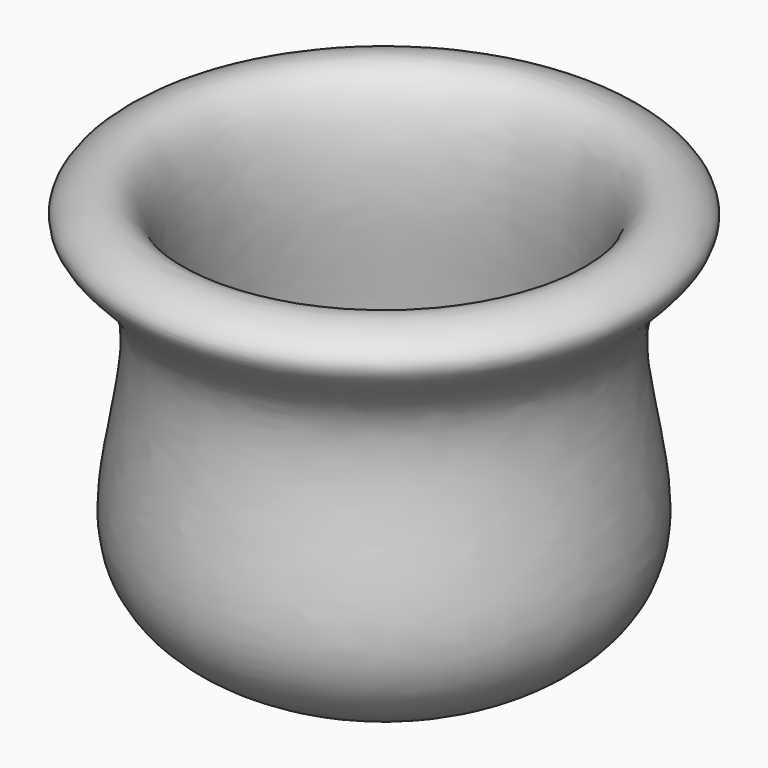
from build123d import *

# Parameters (mm, degrees)
F2_DEPTH     = 12.7
F3_TEXT_SIZE = 10.604480109
F4_DEPTH     = 2.54
F5_DEPTH     = 47.6231673125


# Not quite as in the source:
# - Text() gives the source's letters only with a copy of the font that has no kerning and outlines rounded to 1/6400 em; it was checked with that copy


with BuildPart() as f1:
    # F0 (on Front) → F1 (revolve)
    with BuildSketch(Plane.XZ):
        with BuildLine():
            Line((0, -57.5682340792), (0, -52.8057340792))
            add(Edge.make_bspline(
                [(0, -52.8057340792), (-6.1928503859, -52.7560618863), (-18.0363898415, -50.2076718076), (-28.7476910911, -38.4442162476), (-21.3083678332, -14.0180926687), (-26.1984900624, 3.2355790572), (-39.2409187195, -3.8064788954), (-22.2002577599, -12.224672825), (-34.497030214, -41.2359395167), (-20.295610355, -54.4050094414), (-6.8783044643, -57.4771651446), (0, -57.5682340792)],
                knots=[0.4995456457, 0.4995456457, 0.4995456457, 0.4995456457, 0.5575535114, 0.6075804673, 0.6768554954, 0.7276208231, 0.7642916628, 0.8114346907, 0.8828027767, 0.9381005996, 1, 1, 1, 1], degree=3))
        make_face()
    revolve(axis=Axis((0, 0, -6.35), (0, 0, -1)))


with BuildPart() as f2:
    # F0 (on Front) → F2 (new body, symmetric)
    with BuildSketch(Plane.XZ):
        with BuildLine():
            add(Edge.make_bspline(
                [(0, -57.5682340792), (0.4077877306, -57.5736331996), (0.8148435353, -57.5736492225), (1.2210391681, -57.5682340792)],
                knots=[0, 0, 0, 0, 0.003669773, 0.003669773, 0.003669773, 0.003669773], degree=3))
            Line((0, -57.5682340792), (-12.7, -57.5682340792))
            Line((-12.7, -57.5682340792), (-12.7, -58.8382340792))
            Line((-12.7, -58.8382340792), (12.7, -58.8382340792))
            Line((12.7, -58.8382340792), (12.7, -57.5682340792))
            Line((12.7, -57.5682340792), (1.2210391681, -57.5682340792))
        make_face()
    extrude(amount=F2_DEPTH, both=True)


with BuildPart() as f4_tool:
    # F3 (on face) → F4 (new body)
    with BuildSketch(Plane(origin=(0, 0, -58.8382340792), x_dir=(1, 0, 0), z_dir=(0, 0, -1))):
        with Locations(Location((5.1204622, 0), (0, 0, -180))):
            Text('M', F3_TEXT_SIZE, font='Open Sans', font_style=FontStyle.BOLD, text_align=(TextAlign.LEFT, TextAlign.BOTTOM))
        with Locations((-4.8664622, 0)):
            Text('M', F3_TEXT_SIZE, font='Open Sans', font_style=FontStyle.BOLD, text_align=(TextAlign.LEFT, TextAlign.BOTTOM))
    extrude(amount=-F4_DEPTH)


with BuildPart() as f1_1:
    add(f1.part)

    # F4: cut by f4_tool
    add(f4_tool.part, mode=Mode.SUBTRACT)


with BuildPart() as f2_1:
    add(f2.part)

    # F4: cut by f4_tool
    add(f4_tool.part, mode=Mode.SUBTRACT)

    # F5 (cut, through all): a face of the model
    f5_faces = [f2_1.faces().sort_by_distance(p)[0] for p in [
        (-6.25282e-05, -12.7, -58.2032989039),
    ]]
    extrude(f5_faces, amount=-F5_DEPTH, mode=Mode.SUBTRACT)


solid = f1_1.part
